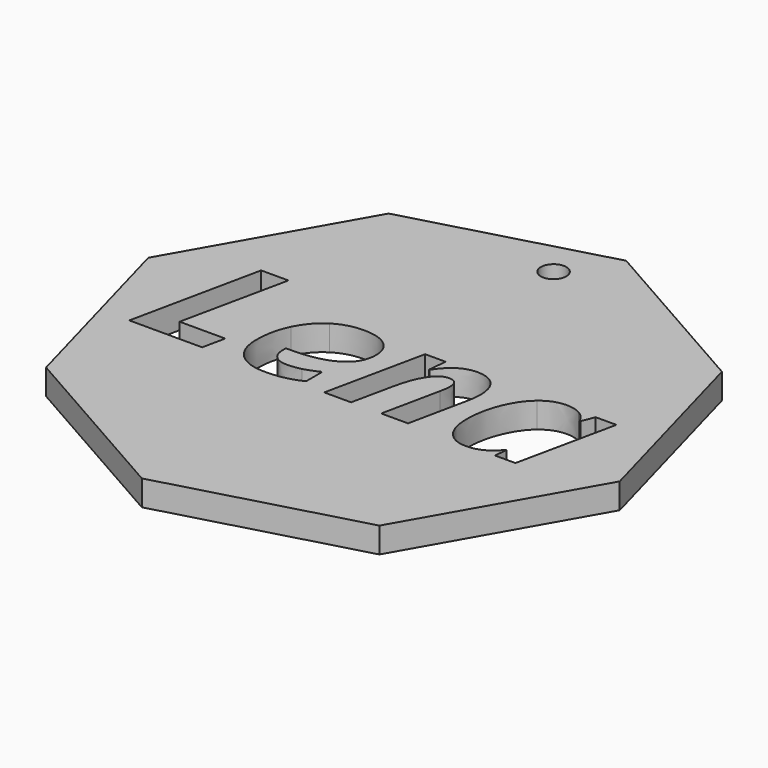
from build123d import *

# Parameters (mm, degrees)
F1_R     = 1.5
F2_DEPTH = 3


with BuildPart() as f2:
    # F1 (on Top) → F2 (new body)
    with BuildSketch(Plane.XY):
        Polygon((19.1138070579, -24.5658658908), (30.8861929421, -3.8551877721), (24.5658658908, 19.1138070579), (3.8551877721, 30.8861929421), (-19.1138070579, 24.5658658908), (-30.8861929421, 3.8551877721), (-24.5658658908, -19.1138070579), (-3.8551877721, -30.8861929421), align=None)
        with BuildLine():
            add(Edge.make_bspline(
                [(-4.1445110049, -6.3067241031), (-5.9517399206, -7.2120212694), (-8.2435888807, -7.2120212694)],
                knots=[0, 0, 0, 1, 1, 1], degree=2))
            add(Edge.make_bspline(
                [(-8.2435888807, -7.2120212694), (-10.4546678333, -7.2120212694), (-11.6746314868, -6.0223463687)],
                knots=[0, 0, 0, 1, 1, 1], degree=2))
            add(Edge.make_bspline(
                [(-11.6746314868, -6.0223463687), (-12.8945951403, -4.832671468), (-12.8945951403, -2.665342936)],
                knots=[0, 0, 0, 1, 1, 1], degree=2))
            add(Edge.make_bspline(
                [(-12.8945951403, -2.665342936), (-12.8945951403, -0.49128357), (-12.0263175607, 1.3024836777)],
                knots=[0, 0, 0, 1, 1, 1], degree=2))
            add(Edge.make_bspline(
                [(-12.0263175607, 1.3024836777), (-11.1580399812, 3.0962509255), (-9.6755738036, 4.03688497)],
                knots=[0, 0, 0, 1, 1, 1], degree=2))
            add(Edge.make_bspline(
                [(-9.6755738036, 4.03688497), (-8.193107626, 4.9775190146), (-6.3219357878, 4.9775190146)],
                knots=[0, 0, 0, 1, 1, 1], degree=2))
            add(Edge.make_bspline(
                [(-6.3219357878, 4.9775190146), (-4.4574947836, 4.9775190146), (-3.4175809383, 4.1210203944)],
                knots=[0, 0, 0, 1, 1, 1], degree=2))
            add(Edge.make_bspline(
                [(-3.4175809383, 4.1210203944), (-2.377667093, 3.2645217742), (-2.377667093, 1.7702766373)],
                knots=[0, 0, 0, 1, 1, 1], degree=2))
            add(Edge.make_bspline(
                [(-2.377667093, 1.7702766373), (-2.377667093, -0.1951268762), (-4.1327320455, -1.2619640573)],
                knots=[0, 0, 0, 1, 1, 1], degree=2))
            add(Edge.make_bspline(
                [(-4.1327320455, -1.2619640573), (-5.887796998, -2.3288012385), (-9.148886047, -2.3288012385)],
                knots=[0, 0, 0, 1, 1, 1], degree=2))
            Line((-9.148886047, -2.3288012385), (-9.687352763, -2.3288012385))
            Line((-9.687352763, -2.3288012385), (-9.7075452649, -2.5509187588))
            Line((-9.7075452649, -2.5509187588), (-9.7075452649, -2.7629400283))
            add(Edge.make_bspline(
                [(-9.7075452649, -2.7629400283), (-9.7075452649, -3.7187184492), (-9.1657131319, -4.2706468331)],
                knots=[0, 0, 0, 1, 1, 1], degree=2))
            add(Edge.make_bspline(
                [(-9.1657131319, -4.2706468331), (-8.6238809989, -4.8225752171), (-7.6142559063, -4.8225752171)],
                knots=[0, 0, 0, 1, 1, 1], degree=2))
            add(Edge.make_bspline(
                [(-7.6142559063, -4.8225752171), (-6.6988624891, -4.8225752171), (-5.9517399206, -4.622332907)],
                knots=[0, 0, 0, 1, 1, 1], degree=2))
            add(Edge.make_bspline(
                [(-5.9517399206, -4.622332907), (-5.2046173521, -4.422090597), (-4.1445110049, -3.9172780508)],
                knots=[0, 0, 0, 1, 1, 1], degree=2))
            Line((-4.1445110049, -3.9172780508), (-4.1445110049, -6.3067241031))
        make_face(mode=Mode.SUBTRACT)
        with BuildLine():
            Line((9.8354311099, -0.2994548025), (8.4354176482, -7))
            Line((8.4354176482, -7), (5.2719256916, -7))
            Line((5.2719256916, -7), (6.712324157, -0.1311839537))
            add(Edge.make_bspline(
                [(6.712324157, -0.1311839537), (6.8805950057, 0.582284445), (6.8805950057, 1.1207511611)],
                knots=[0, 0, 0, 1, 1, 1], degree=2))
            add(Edge.make_bspline(
                [(6.8805950057, 1.1207511611), (6.8805950057, 2.4130712795), (5.7430840681, 2.4130712795)],
                knots=[0, 0, 0, 1, 1, 1], degree=2))
            add(Edge.make_bspline(
                [(5.7430840681, 2.4130712795), (4.7772093962, 2.4130712795), (3.9880191156, 1.2133001279)],
                knots=[0, 0, 0, 1, 1, 1], degree=2))
            add(Edge.make_bspline(
                [(3.9880191156, 1.2133001279), (3.1988288349, 0.0135289762), (2.7478629602, -2.1302416369)],
                knots=[0, 0, 0, 1, 1, 1], degree=2))
            Line((2.7478629602, -2.1302416369), (1.7146799488, -7))
            Line((1.7146799488, -7), (-1.4488120078, -7))
            Line((-1.4488120078, -7), (1.0415965538, 4.7587669112))
            Line((1.0415965538, 4.7587669112), (3.461331359, 4.7587669112))
            Line((3.461331359, 4.7587669112), (3.2392138386, 2.5813421283))
            Line((3.2392138386, 2.5813421283), (3.3031567611, 2.5813421283))
            add(Edge.make_bspline(
                [(3.3031567611, 2.5813421283), (4.8377869018, 4.9775190146), (7.0387696036, 4.9775190146)],
                knots=[0, 0, 0, 1, 1, 1], degree=2))
            add(Edge.make_bspline(
                [(7.0387696036, 4.9775190146), (8.4892643198, 4.9775190146), (9.283502726, 4.1008278926)],
                knots=[0, 0, 0, 1, 1, 1], degree=2))
            add(Edge.make_bspline(
                [(9.283502726, 4.1008278926), (10.0777411321, 3.2241367705), (10.0777411321, 1.5919095376)],
                knots=[0, 0, 0, 1, 1, 1], degree=2))
            add(Edge.make_bspline(
                [(10.0777411321, 1.5919095376), (10.0777411321, 0.8245944673), (9.8354311099, -0.2994548025)],
                knots=[0, 0, 0, 1, 1, 1], degree=2))
        make_face(mode=Mode.SUBTRACT)
        with BuildLine():
            add(Edge.make_bspline(
                [(18.7975365148, -5.4754661103), (17.3874268022, -7.2120212694), (15.4422157905, -7.2120212694)],
                knots=[0, 0, 0, 1, 1, 1], degree=2))
            add(Edge.make_bspline(
                [(15.4422157905, -7.2120212694), (13.894123982, -7.2120212694), (13.0056539005, -6.0913374167)],
                knots=[0, 0, 0, 1, 1, 1], degree=2))
            add(Edge.make_bspline(
                [(13.0056539005, -6.0913374167), (12.1171838191, -4.970653564), (12.1171838191, -2.9514033789)],
                knots=[0, 0, 0, 1, 1, 1], degree=2))
            add(Edge.make_bspline(
                [(12.1171838191, -2.9514033789), (12.1171838191, -0.8682102713), (12.8744026385, 1.0197886518)],
                knots=[0, 0, 0, 1, 1, 1], degree=2))
            add(Edge.make_bspline(
                [(12.8744026385, 1.0197886518), (13.6316214579, 2.9077875749), (14.8633640708, 3.9426532947)],
                knots=[0, 0, 0, 1, 1, 1], degree=2))
            add(Edge.make_bspline(
                [(14.8633640708, 3.9426532947), (16.0951066837, 4.9775190146), (17.5657939019, 4.9775190146)],
                knots=[0, 0, 0, 1, 1, 1], degree=2))
            add(Edge.make_bspline(
                [(17.5657939019, 4.9775190146), (18.5855152453, 4.9775190146), (19.3275896884, 4.5366493909)],
                knots=[0, 0, 0, 1, 1, 1], degree=2))
            add(Edge.make_bspline(
                [(19.3275896884, 4.5366493909), (20.0696641314, 4.0957797671), (20.4802450024, 3.2544255233)],
                knots=[0, 0, 0, 1, 1, 1], degree=2))
            Line((20.4802450024, 3.2544255233), (20.5643804267, 3.2544255233))
            Line((20.5643804267, 3.2544255233), (21.1634246483, 4.7587669112))
            Line((21.1634246483, 4.7587669112), (23.6033519553, 4.7587669112))
            Line((23.6033519553, 4.7587669112), (21.0994817258, -7))
            Line((21.0994817258, -7), (18.6898431716, -7))
            Line((18.6898431716, -7), (18.8379215185, -5.4754661103))
            Line((18.8379215185, -5.4754661103), (18.7975365148, -5.4754661103))
        make_face(mode=Mode.SUBTRACT)
        Polygon((-15.8494312445, -7), (-24.4413407821, -7), (-21.1937134011, 8.3765901595), (-17.9730093559, 8.3765901595), (-20.665342936, -4.3076664199), (-15.2806757757, -4.3076664199), align=None, mode=Mode.SUBTRACT)
        with Locations((0, 25)):
            Circle(F1_R, mode=Mode.SUBTRACT)
    extrude(amount=F2_DEPTH)


solid = f2.part
